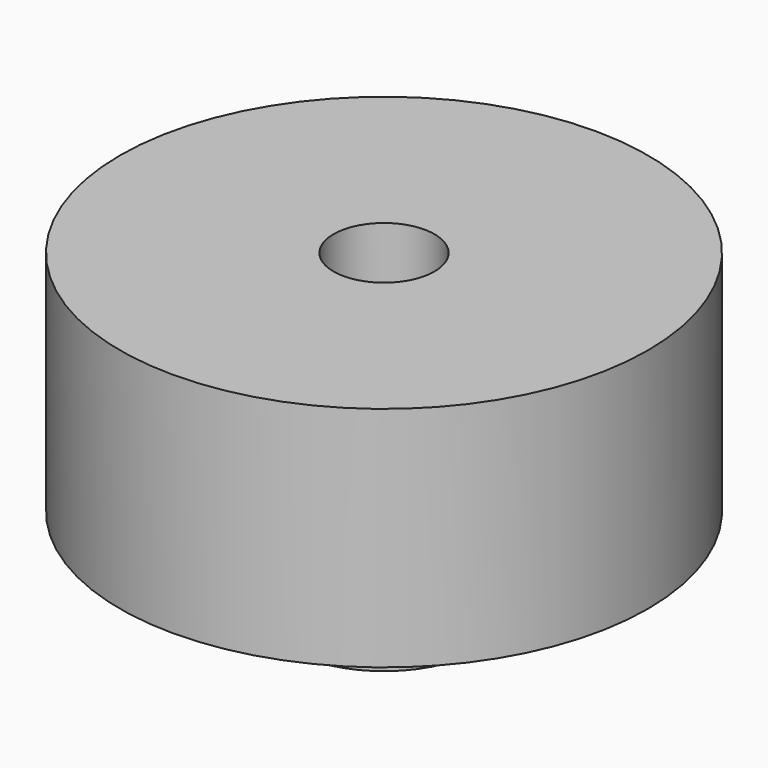
from build123d import *

# Parameters (mm, degrees)
F0_R     = 29
F1_DEPTH = 25
F2_R     = 10.5
F3_DEPTH = 10
F5_D     = 11.1
F9_D     = 2.5
F13_D    = 2.5


with BuildPart() as f1:
    # F0 (on Top) → F1 (new body)
    with BuildSketch(Plane.XY):
        Circle(F0_R)
    extrude(amount=F1_DEPTH)

    # F2 (on face) → F3 (join)
    with BuildSketch(Plane(origin=(0, 0, 0), x_dir=(1, 0, 0), z_dir=(0, 0, -1))):
        Circle(F2_R)
    extrude(amount=F3_DEPTH)

    # F5 (through all)
    with Locations(Plane(origin=(0, 0, -10), x_dir=(1, 0, 0), z_dir=(0, 0, -1))):
        with Locations((0, 0)):
            Hole(F5_D / 2)

    # F9 (through all)
    with Locations(Plane(origin=(-10.5, 0, 0), x_dir=(0, -1, 0), z_dir=(-1, 0, 0))):
        with Locations((0, -5.3152111359)):
            Hole(F9_D / 2)

    # F13 (through all)
    with Locations(Plane(origin=(0, 10.5, 0), x_dir=(-1, 0, 0), z_dir=(0, 1, 0))):
        with Locations((0, -4.9469849671)):
            Hole(F13_D / 2)


solid = f1.part
